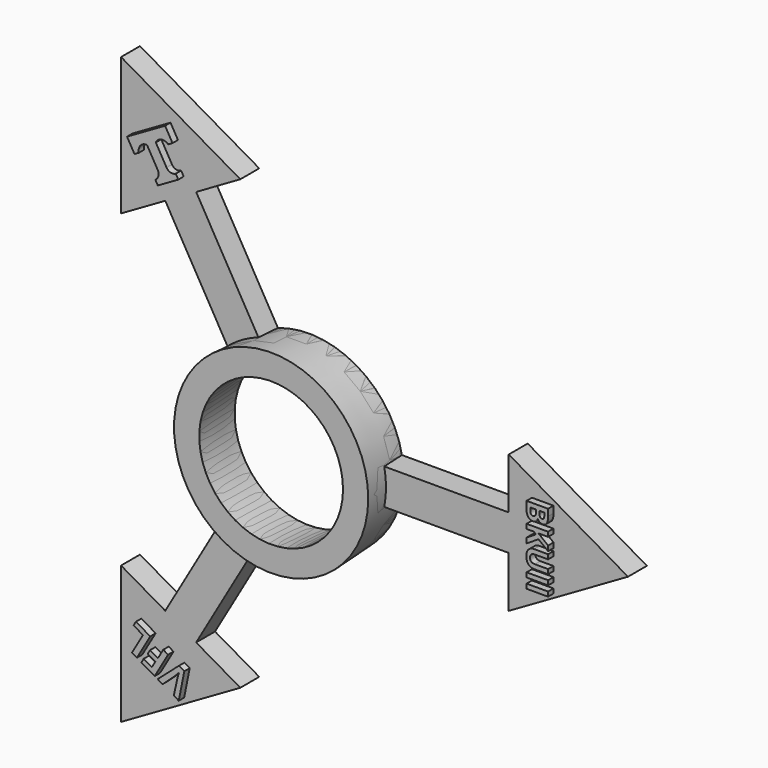
from build123d import *

# Parameters (mm, degrees)
F0_R         = 14
F0_R_2       = 11
F1_DEPTH     = 7
F1_TAPER     = -3
F3_DEPTH     = 3.5
F4_COUNT     = 3
F5_TEXT_SIZE = 4.449970426
F6_DEPTH     = 1


# Not quite as in the source:
# - Text() gives the source's letters only with a copy of the font that has no kerning and outlines rounded to 1/6400 em; it was checked with that copy


with BuildPart() as f1:
    # F0 (on Front) → F1 (new body)
    with BuildSketch(Plane.XZ):
        Circle(F0_R)
        Circle(F0_R_2, mode=Mode.SUBTRACT)
    extrude(amount=F1_DEPTH, taper=F1_TAPER)

    # F2 (on Front) → F3 (join)
    with BuildSketch(Plane.XZ):
        with BuildLine():
            Line((13.7494678476, -2.636689953), (32.3552267201, -2.636689953))
            Line((32.3552267201, -2.636689953), (32.3552267201, 2.636689953))
            Line((32.3552267201, 2.636689953), (13.7494678476, 2.636689953))
            ThreePointArc((13.7494678476, 2.636689953), (13.9372262281, 1.32428285), (14, 0))
            ThreePointArc((14, 0), (13.9372262281, -1.32428285), (13.7494678476, -2.636689953))
        make_face()
        Polygon((32.3552267201, -10.1872146029), (50, 0), (32.3552267201, 10.1872146029), (32.3552267201, 2.636689953), (32.3552267201, -2.636689953), align=None)
    extrude(amount=F3_DEPTH)


with BuildPart() as f4_1:
    # F4: instance of F1
    add(f1.part.rotate(Axis((0, -7, 0), (0, 1, 0)), 1 * 360 / F4_COUNT))


with BuildPart() as f4_2:
    # F4: instance of F1
    add(f1.part.rotate(Axis((0, -7, 0), (0, 1, 0)), 2 * 360 / F4_COUNT))


with BuildPart() as f6:
    # F5 (on face) → F6 (new body)
    with BuildSketch(Plane.XZ.offset(3.5)):
        with BuildLine():
            Line((-18.7655444566, 29.0028764306), (-17.25, 29.8778764306))
            Line((-17.25, 29.8778764306), (-20.5, 35.5070415552))
            Line((-20.5, 35.5070415552), (-23.3145825623, 33.8820415552))
            Line((-23.3145825623, 33.8820415552), (-22.2145825623, 31.9767856668))
            Line((-22.2145825623, 31.9767856668), (-21.5650635095, 32.3517856668))
            ThreePointArc((-21.5650635095, 32.3517856668), (-21.3326003807, 33.3744985304), (-20.3568907413, 33.7591690481))
            Line((-20.3568907413, 33.7591690481), (-18.7745190528, 31.0184208872))
            ThreePointArc((-18.7745190528, 31.0184208872), (-18.6746186303, 30.2596018421), (-19.1405444566, 29.6523954834))
            Line((-19.1405444566, 29.6523954834), (-18.7655444566, 29.0028764306))
        make_face()
        with BuildLine():
            Line((-20.5, 35.5070415552), (-17.25, 29.8778764306))
            Line((-17.25, 29.8778764306), (-15.7344555434, 30.7528764306))
            Line((-15.7344555434, 30.7528764306), (-16.1094555434, 31.4023954834))
            ThreePointArc((-16.1094555434, 31.4023954834), (-16.8682745885, 31.3024950609), (-17.4754809472, 31.7684208872))
            Line((-17.4754809472, 31.7684208872), (-19.0578526356, 34.5091690481))
            ThreePointArc((-19.0578526356, 34.5091690481), (-18.2368633756, 35.1618231237), (-17.2349364905, 34.8517856668))
            Line((-17.2349364905, 34.8517856668), (-16.5854174377, 35.2267856668))
            Line((-16.5854174377, 35.2267856668), (-17.6854174377, 37.1320415552))
            Line((-17.6854174377, 37.1320415552), (-20.5, 35.5070415552))
        make_face()
        Polygon((-18.7425074677, -32.5584613064), (-18.7838541667, -32.5345897786), (-19.1271701389, -33.1292304856), (-19.0858234399, -33.1531020133), (-19.5971081621, -34.0386731294), (-19.6384548611, -34.0148016016), (-19.9830729167, -34.611697583), (-19.2253006884, -35.049197583), (-17.2422277717, -31.6144145362), (-17.958653301, -31.200786064), align=None)
        Polygon((-19.1271701389, -33.1292304856), (-18.7838541667, -32.5345897786), (-19.9077326204, -31.8857182509), (-20.2510485926, -32.4803589578), align=None)
        Polygon((-19.0858234399, -33.1531020133), (-19.1271701389, -33.1292304856), (-19.6384548611, -34.0148016016), (-19.5971081621, -34.0386731294), align=None)
        Polygon((-19.9830729167, -34.611697583), (-19.6384548611, -34.0148016016), (-20.8495372617, -33.3155828516), (-21.1941553173, -33.912478833), align=None)
        with Locations(Location((35.7960212933, 6.0721237078), (0, 0, -90))):
            Text('BKUII', F5_TEXT_SIZE, font='Open Sans', font_style=FontStyle.BOLD, text_align=(TextAlign.LEFT, TextAlign.BOTTOM))
        with BuildLine():
            Line((-18.7930397446, -35.2987635552), (-18.0578202612, -35.7232427219))
            Line((-18.0578202612, -35.7232427219), (-16.2274279224, -34.0546463045))
            add(Edge.make_bspline(
                [(-15.6141328097, -33.4003741203), (-15.7650103176, -33.6009377408), (-16.2274279224, -34.0546463045)],
                knots=[0, 0, 0, 1, 1, 1], degree=2))
            add(Edge.make_bspline(
                [(-15.7358581453, -33.7761391417), (-15.654854635, -33.5021563906), (-15.6141328097, -33.4003741203)],
                knots=[0, 0, 0, 1, 1, 1], degree=2))
            add(Edge.make_bspline(
                [(-15.8680875205, -34.2621115822), (-15.8168616556, -34.0501218927), (-15.7358581453, -33.7761391417)],
                knots=[0, 0, 0, 1, 1, 1], degree=2))
            Line((-15.8680875205, -34.2621115822), (-16.4016970281, -36.6794059164))
            Line((-16.4016970281, -36.6794059164), (-15.6664775447, -37.103885083))
            Line((-15.6664775447, -37.103885083), (-14.8486297807, -32.9963589807))
            Line((-14.8486297807, -32.9963589807), (-15.6424864008, -32.5380256474))
            Line((-15.6424864008, -32.5380256474), (-18.7930397446, -35.2987635552))
        make_face()
        Polygon((-21.866227115, -33.5244579997), (-19.8831541983, -30.0896749529), (-22.0046157343, -28.864848564), (-22.3518379566, -29.4662550944), (-20.9588300805, -30.2705085666), (-22.594680775, -33.103885083), align=None)
    extrude(amount=F6_DEPTH)


solid = Compound([f1.part, f4_1.part, f4_2.part, f6.part])
